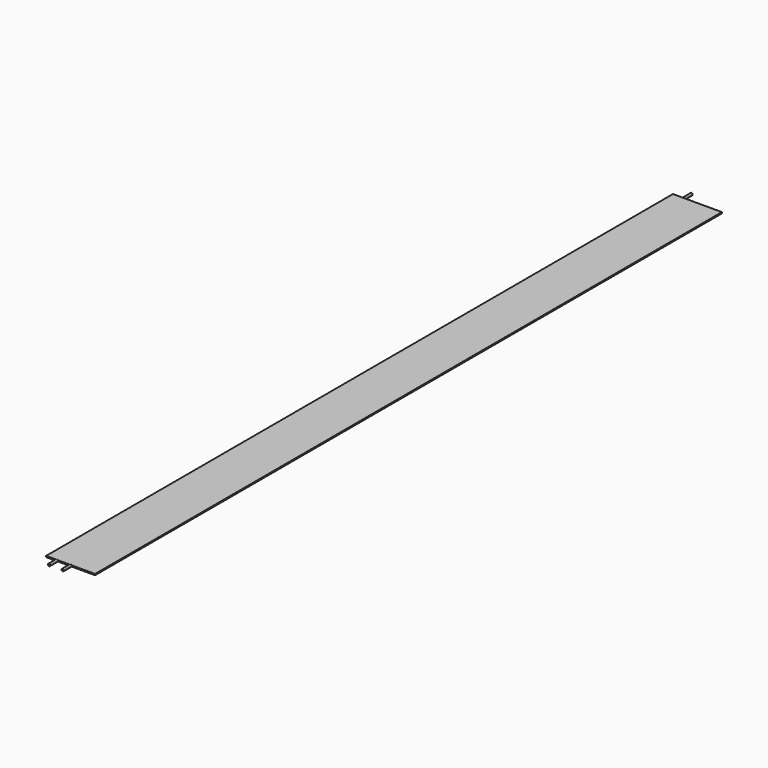
from build123d import *

# Parameters (mm, degrees)
F1_DEPTH = 3
F3_DEPTH = 25
F5_DEPTH = 25
F7_DEPTH = 25


# Not quite as in the source:
# - a feature names something its author has since deleted; it is built from what else it names


with BuildPart() as f1:
    # F0 (on Top) → F1 (new body)
    with BuildSketch(Plane.XY):
        Polygon((-5, 1855.804875493), (-30, 1855.804875493), (-30, -144.195124507), (-5, -144.195124507), (-5, -164.195124507), (0, -164.195124507), (0, -144.195124507), (30, -144.195124507), (30, -164.195124507), (35, -164.195124507), (35, -144.195124507), (95, -144.195124507), (95, 1855.804875493), (0, 1855.804875493), (0, 1875.804875493), (-5, 1875.804875493), align=None)
    extrude(amount=F1_DEPTH)

    # F2 (on face) → F3 (join)
    with BuildSketch(Plane.XZ.offset(144.195124507)):
        with BuildLine():
            Line((35, 3), (35.0980762114, 3))
            ThreePointArc((35.0980762114, 3), (29.5, 1.5), (35.0980762114, 0))
            Line((35.0980762114, 0), (35, 0))
            Line((35, 0), (35, 3))
        make_face()
        with BuildLine():
            ThreePointArc((35.0980762114, 0), (35.3977774789, 0.7235428647), (35.5, 1.5))
            ThreePointArc((35.5, 1.5), (35.3977774789, 2.2764571353), (35.0980762114, 3))
            Line((35.0980762114, 3), (35, 3))
            Line((35, 3), (35, 0))
            Line((35, 0), (35.0980762114, 0))
        make_face()
    extrude(amount=F3_DEPTH)

    # F4 (on face) → F5 (join)
    with BuildSketch(Plane(origin=(0, 1855.804875493, 0), x_dir=(-1, 0, 0), z_dir=(0, 1, 0))):
        with BuildLine():
            Line((0, 3), (-0.0980762114, 3))
            ThreePointArc((-0.0980762114, 3), (-0.5, 1.5), (-0.0980762114, 0))
            Line((-0.0980762114, 0), (0, 0))
            Line((0, 0), (0, 3))
        make_face()
        with BuildLine():
            ThreePointArc((-0.0980762114, 0), (3.2764571353, -1.3977774789), (5.5, 1.5))
            ThreePointArc((5.5, 1.5), (3.2764571353, 4.3977774789), (-0.0980762114, 3))
            Line((-0.0980762114, 3), (0, 3))
            Line((0, 3), (0, 0))
            Line((0, 0), (-0.0980762114, 0))
        make_face()
    extrude(amount=F5_DEPTH)

    # F6 (on face) → F7 (join)
    with BuildSketch(Plane.XZ.offset(144.195124507)):
        with BuildLine():
            ThreePointArc((0.0783741164, 0), (0.3926737069, 0.7383586703), (0.5, 1.5336188953))
            ThreePointArc((0.5, 1.5336188953), (0.4027223964, 2.2913805262), (0.1171982072, 3))
            Line((0.1171982072, 3), (0, 3))
            Line((0, 3), (0, 0))
            Line((0, 0), (0.0783741164, 0))
        make_face()
        with BuildLine():
            Line((0, 3), (0.1171982072, 3))
            ThreePointArc((0.1171982072, 3), (-5.4997488132, 1.5724397355), (0.0783741164, 0))
            Line((0.0783741164, 0), (0, 0))
            Line((0, 0), (0, 3))
        make_face()
    extrude(amount=F7_DEPTH)


solid = f1.part
